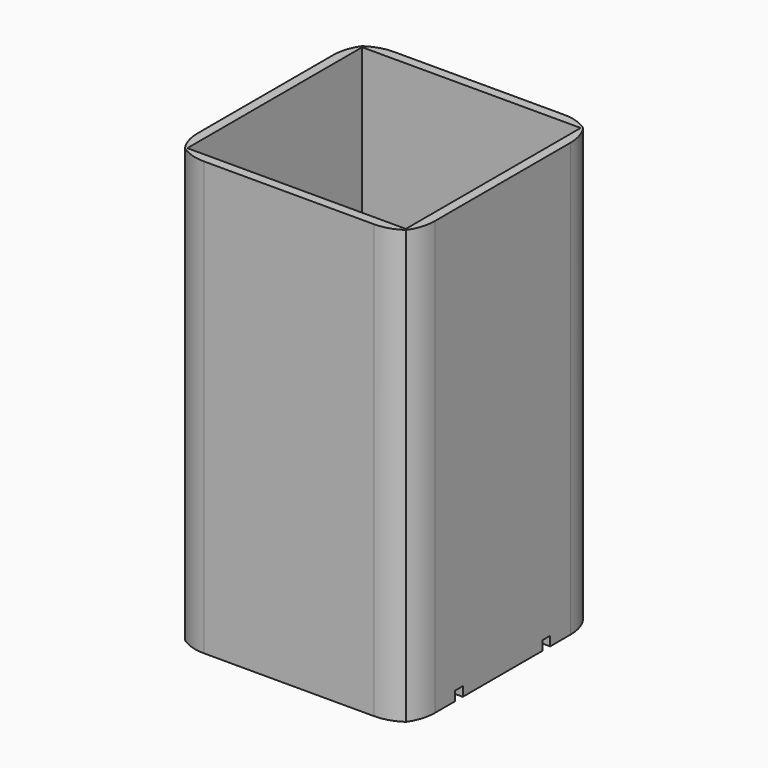
from build123d import *

# Parameters (mm, degrees)
F0_W        = 80.0557104707
F0_H        = 80.0557104707
F0_W_2      = 73.7057104707
F0_H_2      = 73.7057104707
F0_W_3      = 39.99992
F0_H_3      = 39.99992
F1_DEPTH    = 6.35
F2_DEPTH    = 9.144
F3_DEPTH    = 139.7
F4_W        = 20.0278952353
F4_H        = 3.175
F5_DEPTH    = 3.175
F7_SIZE     = 5.08
F6_T1_DEPTH = 177.6130734528


# Not quite as in the source:
# - a fillet or chamfer that OpenCascade refuses, or shapes differently, is made with other operations: its cross-section is extruded or revolved along the edge and cut away or added


with BuildPart() as f1:
    # F0 (on Top) → F1 (new body)
    with BuildSketch(Plane.XY):
        Rectangle(F0_W, F0_H)
        Rectangle(F0_W_2, F0_H_2, mode=Mode.SUBTRACT)
        Rectangle(F0_W_2, F0_H_2)
        Rectangle(F0_W_3, F0_H_3, mode=Mode.SUBTRACT)
        Rectangle(F0_W_3, F0_H_3)
    extrude(amount=-F1_DEPTH)

    # F0 (on Top) → F2 (cut)
    with BuildSketch(Plane.XY):
        Rectangle(F0_W_3, F0_H_3)
    extrude(amount=-F2_DEPTH, mode=Mode.SUBTRACT)

    # F0 (on Top) → F3 (join)
    with BuildSketch(Plane.XY):
        Rectangle(F0_W, F0_H)
        Rectangle(F0_W_2, F0_H_2, mode=Mode.SUBTRACT)
    extrude(amount=F3_DEPTH)

    # F4 (on face) → F5 (cut)
    with BuildSketch(Plane(origin=(0, 0, -6.35), x_dir=(1, 0, 0), z_dir=(0, 0, -1))):
        with Locations((30.0139076177, 18.41246)):
            Rectangle(F4_W, F4_H)
        with Locations((30.0139076177, -18.41246)):
            Rectangle(F4_W, F4_H)
    extrude(amount=-F5_DEPTH, mode=Mode.SUBTRACT)

    # F7
    f7_edges = [f1.edges().sort_by_distance(p)[0] for p in [
        (40.027855, -40.027855, 66.675),
        (-40.027855, -40.027855, 66.675),
        (-40.027855, 40.027855, 66.675),
        (40.027855, 40.027855, 66.675),
    ]]
    chamfer(f7_edges, length=F7_SIZE)

    # F6: fillet of radius 15.24 on 8 edges, made by hand

    # F6_s2 → F6_t1 (cut)
    with BuildSketch(Plane.XY.offset(-22.1315367264)):
        with BuildLine():
            ThreePointArc((-28.6352405448, -40.0278552353), (-34.467336054, -38.8677793108), (-39.4115478901, -35.5641625806))
            Line((-39.4115478901, -35.5641625806), (-34.9478552353, -40.0278552353))
            Line((-34.9478552353, -40.0278552353), (-28.6352405448, -40.0278552353))
        make_face()
        with BuildLine():
            ThreePointArc((-35.5641625806, -39.4115478901), (-38.8677793108, -34.467336054), (-40.0278552353, -28.6352405448))
            Line((-40.0278552353, -28.6352405448), (-40.0278552353, -34.9478552353))
            Line((-40.0278552353, -34.9478552353), (-35.5641625806, -39.4115478901))
        make_face()
        with BuildLine():
            ThreePointArc((-35.5641625806, 39.4115478901), (-38.8677793108, 34.467336054), (-40.0278552353, 28.6352405448))
            Line((-40.0278552353, 28.6352405448), (-40.0278552353, 34.9478552353))
            Line((-40.0278552353, 34.9478552353), (-35.5641625806, 39.4115478901))
        make_face()
        with BuildLine():
            ThreePointArc((-28.6352405448, 40.0278552353), (-34.467336054, 38.8677793108), (-39.4115478901, 35.5641625806))
            Line((-39.4115478901, 35.5641625806), (-34.9478552353, 40.0278552353))
            Line((-34.9478552353, 40.0278552353), (-28.6352405448, 40.0278552353))
        make_face()
        with BuildLine():
            ThreePointArc((40.0278552353, -28.6352405448), (38.8677793108, -34.467336054), (35.5641625806, -39.4115478901))
            Line((35.5641625806, -39.4115478901), (40.0278552353, -34.9478552353))
            Line((40.0278552353, -34.9478552353), (40.0278552353, -28.6352405448))
        make_face()
        with BuildLine():
            ThreePointArc((39.4115478901, -35.5641625806), (34.467336054, -38.8677793108), (28.6352405448, -40.0278552353))
            Line((28.6352405448, -40.0278552353), (34.9478552353, -40.0278552353))
            Line((34.9478552353, -40.0278552353), (39.4115478901, -35.5641625806))
        make_face()
        with BuildLine():
            ThreePointArc((40.0278552353, 28.6352405448), (38.8677793108, 34.467336054), (35.5641625806, 39.4115478901))
            Line((35.5641625806, 39.4115478901), (40.0278552353, 34.9478552353))
            Line((40.0278552353, 34.9478552353), (40.0278552353, 28.6352405448))
        make_face()
        with BuildLine():
            ThreePointArc((39.4115478901, 35.5641625806), (34.467336054, 38.8677793108), (28.6352405448, 40.0278552353))
            Line((28.6352405448, 40.0278552353), (34.9478552353, 40.0278552353))
            Line((34.9478552353, 40.0278552353), (39.4115478901, 35.5641625806))
        make_face()
    extrude(amount=F6_T1_DEPTH, mode=Mode.SUBTRACT)


solid = f1.part
